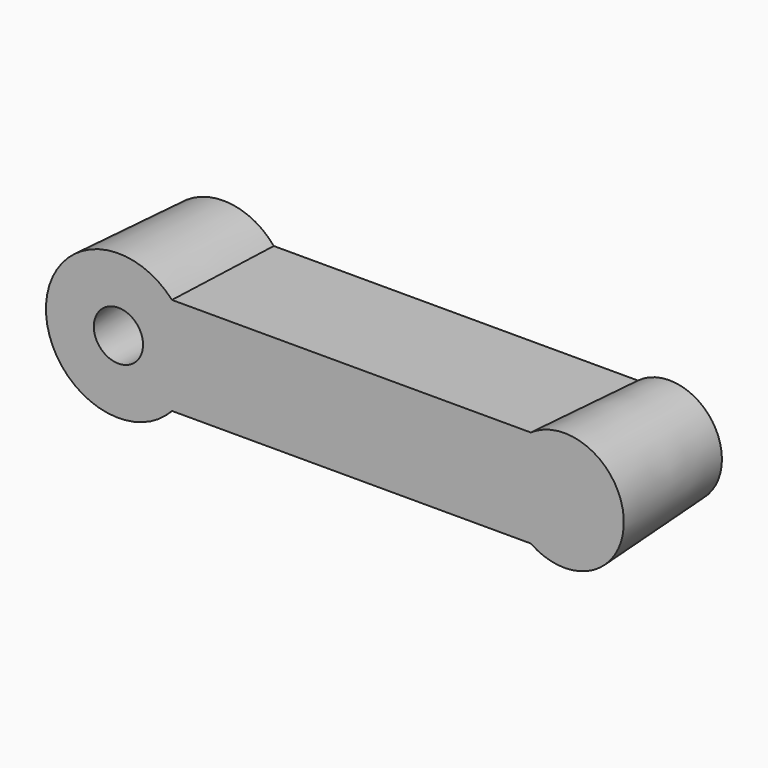
from build123d import *

# Parameters (mm, degrees)
F0_R                   = 6
F1_DEPTH               = 25
DRAFT_F1_DRAFTED_ANGLE = -3


# Not quite as in the source:
# - an extrude with a draft is written as a straight extrude whose walls are then drafted


with BuildPart() as f1:
    # F0 (on Front) → F1 (new body)
    with BuildSketch(Plane.XZ):
        with BuildLine():
            ThreePointArc((-11.7776124479, -8), (-9.6283935073, -4.2539052968), (-8.8822988041, 0))
            ThreePointArc((-8.8822988041, 0), (-9.6283935073, 4.2539052968), (-11.7776124479, 8))
            ThreePointArc((-11.7776124479, 8), (-33.8822988041, 0), (-11.7776124479, -8))
        make_face()
        with Locations((-21.3822988041, 0)):
            Circle(F0_R, mode=Mode.SUBTRACT)
        with BuildLine():
            ThreePointArc((-11.7776124479, 8), (-9.6283935073, 4.2539052968), (-8.8822988041, 0))
            ThreePointArc((-8.8822988041, 0), (-9.6283935073, -4.2539052968), (-11.7776124479, -8))
            Line((-11.7776124479, -8), (57.6177011959, -8))
            ThreePointArc((57.6177011959, -8), (53.6177011959, 0), (57.6177011959, 8))
            Line((57.6177011959, 8), (-11.7776124479, 8))
        make_face()
        with BuildLine():
            ThreePointArc((73.6177011959, 0), (68.0898371509, 8.94427191), (57.6177011959, 8))
            ThreePointArc((57.6177011959, 8), (53.6177011959, 0), (57.6177011959, -8))
            ThreePointArc((57.6177011959, -8), (68.0898371509, -8.94427191), (73.6177011959, 0))
        make_face()
    extrude(amount=F1_DEPTH)

    # draft_F1_drafted
    draft_f1_drafted_walls = [f1.faces().sort_by_distance(p)[0] for p in [
        (-33.8822988041, -16.6666666667, 0),
        (22.920044374, -16.6666666667, -8),
        (73.6177011959, -16.6666666667, 0),
        (22.920044374, -16.6666666667, 8),
        (-27.3822988041, -16.6666666667, 0),
    ]]
    draft(draft_f1_drafted_walls, neutral_plane=Plane.XZ, angle=DRAFT_F1_DRAFTED_ANGLE)


solid = f1.part
